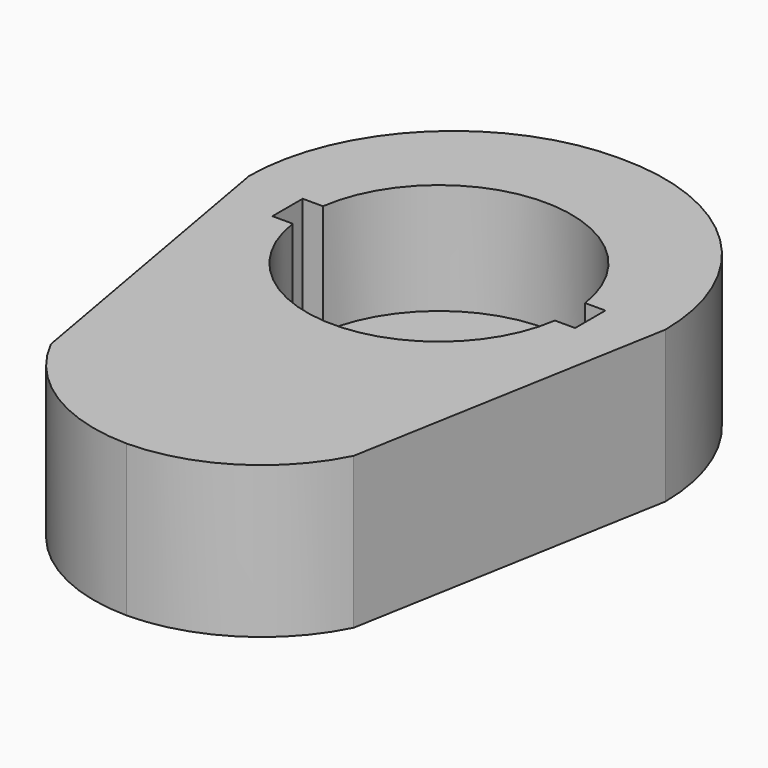
from build123d import *

# Parameters (mm, degrees)
F1_DEPTH = 12.7
F2_R     = 3.175
F3_DEPTH = 9.3
F4_DEPTH = 25.4


# Not quite as in the source:
# - ends of sketch curves that miss each other by under 0.0002 mm in the source are joined


with BuildPart() as f1:
    # F0 (on Top) → F1 (new body)
    with BuildSketch(Plane.XY):
        with BuildLine():
            ThreePointArc((0, -32.75), (7.4692491087, -30.572048574), (12.7, -24.8125))
            Line((12.7, -24.8125), (17.4625, 1.9280540291))
            ThreePointArc((17.4625, 1.9280540291), (12.2942741687, 14.1229194267), (0, 19.05))
            ThreePointArc((0, 19.05), (-12.2942741687, 14.1229194267), (-17.4625, 1.9280540291))
            Line((-17.4625, 1.9280540291), (-12.7, -24.8125))
            ThreePointArc((-12.7, -24.8125), (-7.4692491087, -30.572048574), (0, -32.75))
        make_face()
    extrude(amount=F1_DEPTH)

    # F2 (on face) → F3 (cut)
    with BuildSketch(Plane.XY.offset(12.7)):
        with BuildLine():
            Line((12.7, 1.5875), (10.9985226281, 1.5875))
            ThreePointArc((10.9985226281, 1.5875), (0, 11.1125), (-10.9985226281, 1.5875))
            Line((-10.9985226281, 1.5875), (-12.7, 1.5875))
            Line((-12.7, 1.5875), (-12.7, 0))
            Line((-12.7, 0), (-12.7, -1.5875))
            Line((-12.7, -1.5875), (-10.9985226281, -1.5875))
            ThreePointArc((-10.9985226281, -1.5875), (0, -11.1125), (10.9985226281, -1.5875))
            Line((10.9985226281, -1.5875), (12.7, -1.5875))
            Line((12.7, -1.5875), (12.7, 0))
            Line((12.7, 0), (12.7, 1.5875))
        make_face()
        Circle(F2_R, mode=Mode.SUBTRACT)
    extrude(amount=-F3_DEPTH, mode=Mode.SUBTRACT)

    # F4 (cut): a face of the model
    f4_faces = [f1.faces().sort_by_distance(p)[0] for p in [
        (0, 0, 12.7),
    ]]
    extrude(f4_faces, amount=-F4_DEPTH, mode=Mode.SUBTRACT)


solid = f1.part
